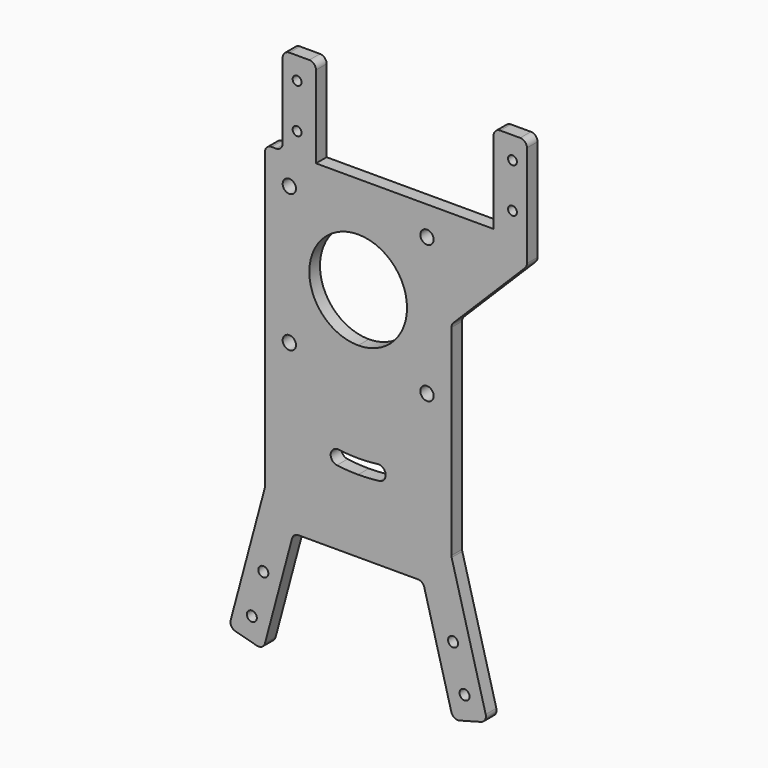
from build123d import *
from build123d import SkipClean  # not in build123d's __all__

# Parameters (mm, degrees)
F1_R     = 1.125
F1_R_2   = 1.5
F2_DEPTH = 3
F4_R     = 1
F4_W     = 7.5
F4_H     = 20
F5_DEPTH = 3
F6_R     = 1.5


with BuildPart() as f2:
    # F1 (on Front) → F2 (new body)
    with BuildSketch(Plane.XZ):
        with BuildLine():
            Line((0, 22), (0, 11))
            ThreePointArc((0, 11), (11, 0), (0, -11))
            Line((0, -11), (0, -33.375))
            ThreePointArc((0, -33.375), (2.1828294381, -33.3035415631), (4.3563116653, -33.0894722484))
            ThreePointArc((4.3563116653, -33.0894722484), (6.1795146274, -34.4884650857), (4.7805217901, -36.3116680478))
            ThreePointArc((4.7805217901, -36.3116680478), (2.3953896081, -36.5465830636), (0, -36.625))
            Line((0, -36.625), (0, -53))
            Line((0, -53), (14.5895357507, -53))
            Line((14.5895357507, -53), (21.3767935231, -78.330390851))
            Line((21.3767935231, -78.330390851), (29.104200163, -76.2598384823))
            Line((29.104200163, -76.2598384823), (21, -46.0145517191))
            Line((21, -46.0145517191), (21, 22))
            Line((21, 22), (0, 22))
        make_face()
        with Locations((21.3582111666, -62.8062272723)):
            Circle(F1_R, mode=Mode.SUBTRACT)
        with Locations((23.9464016176, -72.4654855352)):
            Circle(F1_R, mode=Mode.SUBTRACT)
        with Locations((15.5, -15.5)):
            Circle(F1_R_2, mode=Mode.SUBTRACT)
        with Locations((15.5, 15.5)):
            Circle(F1_R_2, mode=Mode.SUBTRACT)
    extrude(amount=F2_DEPTH)

    # F3: F2 across face


with BuildPart() as f2_1:
    add(f2.part, clean=False)
    with SkipClean():  # cleaning this boolean's faces spoils the solid; the shape is the same uncleaned
        add(f2.part.mirror(Plane(origin=(0, -1.5, -22.1875), x_dir=(0, -1, 0), z_dir=(-1, 0, 0))), clean=False)

    # F4 (on Front) → F5 (join)
    with BuildSketch(Plane.XZ):
        Polygon((38, 17), (38, 42), (30.5, 42), (30.5, 22), (21, 22), (21, 0), align=None)
        with Locations((34.75, 27)):
            Circle(F4_R, mode=Mode.SUBTRACT)
        with Locations((34.75, 37)):
            Circle(F4_R, mode=Mode.SUBTRACT)
        with Locations((-13.25, 32)):
            Rectangle(F4_W, F4_H)
        with Locations((-13.75, 27)):
            Circle(F4_R, mode=Mode.SUBTRACT)
        with Locations((-13.75, 37)):
            Circle(F4_R, mode=Mode.SUBTRACT)
    extrude(amount=F5_DEPTH)

    # F6
    f6_edges = [f2_1.edges().sort_by_distance(p)[0] for p in [
        (-21, -1.5, 22),
        (-17, -1.5, 42),
        (-9.5, -1.5, 42),
        (30.5, -1.5, 42),
        (38, -1.5, 42),
        (38, -1.5, 17),
        (21, -1.5, 0),
        (21, -1.5, -46.014552),
        (29.1042, -1.5, -76.259838),
        (21.376794, -1.5, -78.330391),
        (-14.589536, -1.5, -53),
        (-21.376794, -1.5, -78.330391),
        (-29.1042, -1.5, -76.259838),
        (14.589536, -1.5, -53),
        (-21, -1.5, -46.014552),
        (-17, -1.5, 22),
    ]]
    fillet(f6_edges, radius=F6_R)


solid = f2_1.part
